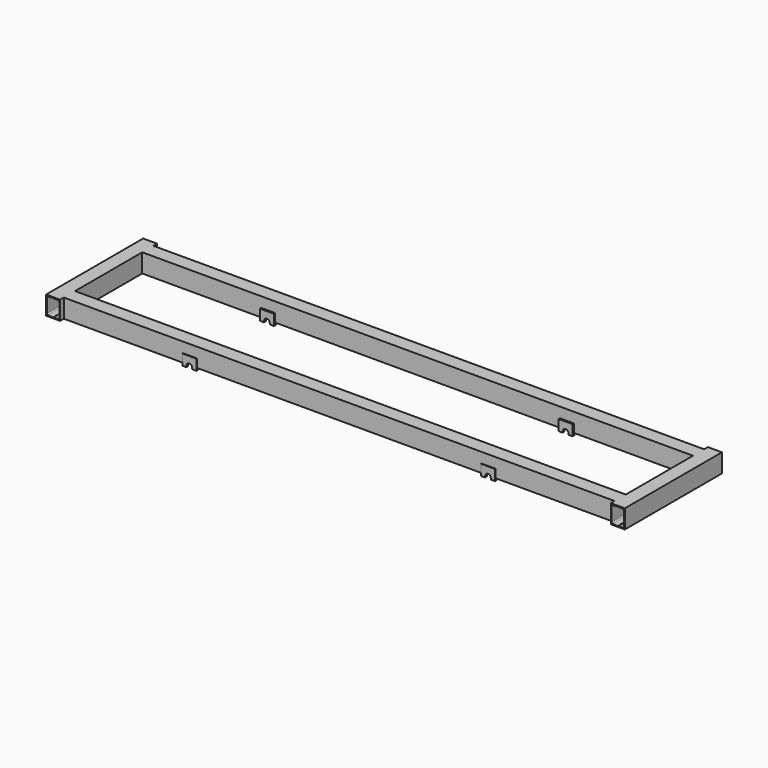
from build123d import *

# Parameters (mm, degrees)
F4_DEPTH       = 3000
F5_W           = 75
F5_H           = 200
F5_W_2         = 50
F5_W_3         = 25
F6_DEPTH       = 1200.001
F8_DEPTH       = 650
F9_W           = 150
F9_H           = 115
F10_DEPTH      = 600
F10_DEPTH_BACK = 600
F11_W          = 370
F11_H          = 130
F11_W_2        = 260
F11_H_2        = 65
F11_W_3        = 110
F11_W_4        = 150
F12_DEPTH      = 50
F13_DEPTH      = 500
F14_DEPTH      = 107.5
F15_DEPTH      = 107.5
F17_DEPTH      = 1257.501
F18_W          = 107.5
F18_H          = 125
F18_W_2        = 42.5
F18_H_2        = 865
F18_H_3        = 82.5
F18_H_4        = 42.5
F18_W_3        = 150
F19_DEPTH      = 115


with BuildPart() as f4:
    # F3 (on Right) → F4 (new body, symmetric)
    with BuildSketch(Plane.YZ):
        with BuildLine():
            ThreePointArc((-530.4770655435, -8.6983562622), (-526.5763359791, -6.7747293194), (-525, -2.7211880737))
            Line((-525, -2.7211880737), (-525, 0))
            Line((-525, 0), (-600, 0))
            Line((-600, 0), (-600, -200))
            Line((-600, -200), (-525, -200))
            Line((-525, -200), (-525, -197.2788119263))
            ThreePointArc((-525, -197.2788119263), (-526.5763359791, -193.2252706806), (-530.4770655435, -191.3016437378))
            Line((-530.4770655435, -191.3016437378), (-586.0229344565, -186.4420099022))
            ThreePointArc((-586.0229344565, -186.4420099022), (-589.9236640209, -184.5183829593), (-591.5, -180.4648417136))
            Line((-591.5, -180.4648417136), (-591.5, -19.5351582864))
            ThreePointArc((-591.5, -19.5351582864), (-589.9236640209, -15.4816170407), (-586.0229344565, -13.5579900978))
            Line((-586.0229344565, -13.5579900978), (-530.4770655435, -8.6983562622))
        make_face()
        with BuildLine():
            Line((-525, 0), (-525, -2.7211880737))
            ThreePointArc((-525, -2.7211880737), (-523.4236640209, -6.7747293194), (-519.5229344565, -8.6983562622))
            Line((-519.5229344565, -8.6983562622), (-463.9770655435, -13.5579900978))
            ThreePointArc((-463.9770655435, -13.5579900978), (-460.0763359791, -15.4816170407), (-458.5, -19.5351582864))
            Line((-458.5, -19.5351582864), (-458.5, -180.4648417136))
            ThreePointArc((-458.5, -180.4648417136), (-460.0763359791, -184.5183829593), (-463.9770655435, -186.4420099022))
            Line((-463.9770655435, -186.4420099022), (-519.5229344565, -191.3016437378))
            ThreePointArc((-519.5229344565, -191.3016437378), (-523.4236640209, -193.2252706806), (-525, -197.2788119263))
            Line((-525, -197.2788119263), (-525, -200))
            Line((-525, -200), (-450, -200))
            Line((-450, -200), (-450, 0))
            Line((-450, 0), (-525, 0))
        make_face()
    extrude(amount=F4_DEPTH, both=True)


with BuildPart() as f4b:
    # F3 (on Right) → F4, piece 2 (new body, symmetric)
    with BuildSketch(Plane.YZ):
        with BuildLine():
            Line((450, -200), (525, -200))
            Line((525, -200), (525, -197.2788119263))
            ThreePointArc((525, -197.2788119263), (523.4236640209, -193.2252706806), (519.5229344565, -191.3016437378))
            Line((519.5229344565, -191.3016437378), (463.9770655435, -186.4420099022))
            ThreePointArc((463.9770655435, -186.4420099022), (460.0763359791, -184.5183829593), (458.5, -180.4648417136))
            Line((458.5, -180.4648417136), (458.5, -19.5351582864))
            ThreePointArc((458.5, -19.5351582864), (460.0763359791, -15.4816170407), (463.9770655435, -13.5579900978))
            Line((463.9770655435, -13.5579900978), (519.5229344565, -8.6983562622))
            ThreePointArc((519.5229344565, -8.6983562622), (523.4236640209, -6.7747293194), (525, -2.7211880737))
            Line((525, -2.7211880737), (525, 0))
            Line((525, 0), (450, 0))
            Line((450, 0), (450, -200))
        make_face()
        with BuildLine():
            Line((525, -197.2788119263), (525, -200))
            Line((525, -200), (600, -200))
            Line((600, -200), (600, 0))
            Line((600, 0), (525, 0))
            Line((525, 0), (525, -2.7211880737))
            ThreePointArc((525, -2.7211880737), (526.5763359791, -6.7747293194), (530.4770655435, -8.6983562622))
            Line((530.4770655435, -8.6983562622), (586.0229344565, -13.5579900978))
            ThreePointArc((586.0229344565, -13.5579900978), (589.9236640209, -15.4816170407), (591.5, -19.5351582864))
            Line((591.5, -19.5351582864), (591.5, -180.4648417136))
            ThreePointArc((591.5, -180.4648417136), (589.9236640209, -184.5183829593), (586.0229344565, -186.4420099022))
            Line((586.0229344565, -186.4420099022), (530.4770655435, -191.3016437378))
            ThreePointArc((530.4770655435, -191.3016437378), (526.5763359791, -193.2252706806), (525, -197.2788119263))
        make_face()
    extrude(amount=F4_DEPTH, both=True)


with BuildPart() as f6_tool:
    # F5 (on face) → F6 (new body, through all)
    with BuildSketch(Plane.XZ.offset(600)):
        with Locations((-3062.5, -100)):
            Rectangle(F5_W, F5_H)
        with Locations((-2975, -100)):
            Rectangle(F5_W_2, F5_H)
        with Locations((3012.5, -100)):
            Rectangle(F5_W_3, F5_H)
        with Locations((2975, -100)):
            Rectangle(F5_W_2, F5_H)
        with Locations((3062.5, -100)):
            Rectangle(F5_W, F5_H)
        with Locations((-3012.5, -100)):
            Rectangle(F5_W_3, F5_H)
    extrude(amount=-F6_DEPTH)


with BuildPart() as f4_1:
    add(f4.part)

    # F6: cut by f6_tool
    add(f6_tool.part, mode=Mode.SUBTRACT)



with BuildPart() as f4b_1:
    add(f4b.part)

    # F6: cut by f6_tool
    add(f6_tool.part, mode=Mode.SUBTRACT)


with BuildPart() as f4_2:
    add(f4_1.part)

    add(f4b_1.part)  # F8 merges F4b
    # F7 (on Front) → F8 (join, symmetric)
    with BuildSketch(Plane.XZ):
        with BuildLine():
            Line((-3100, -200), (-3025, -200))
            Line((-3025, -200), (-3025, -197.2788119263))
            ThreePointArc((-3025, -197.2788119263), (-3026.5763359791, -193.2252706806), (-3030.4770655435, -191.3016437378))
            Line((-3030.4770655435, -191.3016437378), (-3081.0022910416, -186.8812592846))
            ThreePointArc((-3081.0022910416, -186.8812592846), (-3088.4786893733, -183.1943076441), (-3091.5, -175.4250202565))
            Line((-3091.5, -175.4250202565), (-3091.5, -24.5749797435))
            ThreePointArc((-3091.5, -24.5749797435), (-3088.4786893733, -16.8056923559), (-3081.0022910416, -13.1187407154))
            Line((-3081.0022910416, -13.1187407154), (-3030.4770655435, -8.6983562622))
            ThreePointArc((-3030.4770655435, -8.6983562622), (-3026.5763359791, -6.7747293194), (-3025, -2.7211880737))
            Line((-3025, -2.7211880737), (-3025, 0))
            Line((-3025, 0), (-3100, 0))
            Line((-3100, 0), (-3100, -200))
        make_face()
        with BuildLine():
            Line((-3025, -200), (-2950, -200))
            Line((-2950, -200), (-2950, 0))
            Line((-2950, 0), (-3025, 0))
            Line((-3025, 0), (-3025, -2.7211880737))
            ThreePointArc((-3025, -2.7211880737), (-3023.4236640209, -6.7747293194), (-3019.5229344565, -8.6983562622))
            Line((-3019.5229344565, -8.6983562622), (-2968.9977089584, -13.1187407154))
            ThreePointArc((-2968.9977089584, -13.1187407154), (-2961.5213106267, -16.8056923559), (-2958.5, -24.5749797435))
            Line((-2958.5, -24.5749797435), (-2958.5, -175.4250202565))
            ThreePointArc((-2958.5, -175.4250202565), (-2961.5213106267, -183.1943076441), (-2968.9977089584, -186.8812592846))
            Line((-2968.9977089584, -186.8812592846), (-3019.5229344565, -191.3016437378))
            ThreePointArc((-3019.5229344565, -191.3016437378), (-3023.4236640209, -193.2252706806), (-3025, -197.2788119263))
            Line((-3025, -197.2788119263), (-3025, -200))
        make_face()
        with BuildLine():
            Line((3025, -2.7211880737), (3025, 0))
            Line((3025, 0), (2950, 0))
            Line((2950, 0), (2950, -200))
            Line((2950, -200), (3025, -200))
            Line((3025, -200), (3025, -197.2788119263))
            ThreePointArc((3025, -197.2788119263), (3023.4236640209, -193.2252706806), (3019.5229344565, -191.3016437378))
            Line((3019.5229344565, -191.3016437378), (2968.9977089584, -186.8812592846))
            ThreePointArc((2968.9977089584, -186.8812592846), (2961.5213106267, -183.1943076441), (2958.5, -175.4250202565))
            Line((2958.5, -175.4250202565), (2958.5, -24.5749797435))
            ThreePointArc((2958.5, -24.5749797435), (2961.5213106267, -16.8056923559), (2968.9977089584, -13.1187407154))
            Line((2968.9977089584, -13.1187407154), (3019.5229344565, -8.6983562622))
            ThreePointArc((3019.5229344565, -8.6983562622), (3023.4236640209, -6.7747293194), (3025, -2.7211880737))
        make_face()
        with BuildLine():
            Line((3100, 0), (3025, 0))
            Line((3025, 0), (3025, -2.7211880737))
            ThreePointArc((3025, -2.7211880737), (3026.5763359791, -6.7747293194), (3030.4770655435, -8.6983562622))
            Line((3030.4770655435, -8.6983562622), (3081.0022910416, -13.1187407154))
            ThreePointArc((3081.0022910416, -13.1187407154), (3088.4786893733, -16.8056923559), (3091.5, -24.5749797435))
            Line((3091.5, -24.5749797435), (3091.5, -175.4250202565))
            ThreePointArc((3091.5, -175.4250202565), (3088.4786893733, -183.1943076441), (3081.0022910416, -186.8812592846))
            Line((3081.0022910416, -186.8812592846), (3030.4770655435, -191.3016437378))
            ThreePointArc((3030.4770655435, -191.3016437378), (3026.5763359791, -193.2252706806), (3025, -197.2788119263))
            Line((3025, -197.2788119263), (3025, -200))
            Line((3025, -200), (3100, -200))
            Line((3100, -200), (3100, 0))
        make_face()
    extrude(amount=F8_DEPTH, both=True)

    # F9 (on Front) → F10 (cut, two sides)
    with BuildSketch(Plane.XZ) as f10_sk:
        with Locations((-1600, -167.5)):
            Rectangle(F9_W, F9_H)
        with Locations((1600, -167.5)):
            Rectangle(F9_W, F9_H)
    extrude(amount=F10_DEPTH, mode=Mode.SUBTRACT)
    extrude(f10_sk.sketch, amount=-F10_DEPTH_BACK, mode=Mode.SUBTRACT)

    # F11 (on face) → F12 (cut)
    with BuildSketch(Plane(origin=(0, 0, -200), x_dir=(1, 0, 0), z_dir=(0, 0, -1))):
        with Locations((-1600, -525)):
            Rectangle(F11_W, F11_H)
        with Locations((1600, -525)):
            Rectangle(F11_W, F11_H)
        with Locations((-1655, 557.5)):
            Rectangle(F11_W_2, F11_H_2)
        with Locations((-1470, 557.5)):
            Rectangle(F11_W_3, F11_H_2)
        with Locations((-1655, 492.5)):
            Rectangle(F11_W_2, F11_H_2)
        with Locations((-1470, 492.5)):
            Rectangle(F11_W_3, F11_H_2)
        with Locations((1470, 557.5)):
            Rectangle(F11_W_3, F11_H_2)
        with Locations((1600, 557.5)):
            Rectangle(F11_W_4, F11_H_2)
        with Locations((1730, 557.5)):
            Rectangle(F11_W_3, F11_H_2)
        with Locations((1730, 492.5)):
            Rectangle(F11_W_3, F11_H_2)
        with Locations((1600, 492.5)):
            Rectangle(F11_W_4, F11_H_2)
        with Locations((1470, 492.5)):
            Rectangle(F11_W_3, F11_H_2)
    extrude(amount=-F12_DEPTH, mode=Mode.SUBTRACT)


with BuildPart() as f13:
    # F9 (on Front) → F13 (new body, symmetric)
    with BuildSketch(Plane.XZ):
        with Locations((-1600, -167.5)):
            Rectangle(F9_W, F9_H)
    extrude(amount=F13_DEPTH, both=True)

    # F14 (add): a face of the model
    f14_faces = [f13.faces().sort_by_distance(p)[0] for p in [
        (-1600, -500, -167.5),
    ]]
    extrude(f14_faces, amount=F14_DEPTH)


with BuildPart() as f13b:
    # F9 (on Front) → F13, piece 2 (new body, symmetric)
    with BuildSketch(Plane.XZ):
        with Locations((1600, -167.5)):
            Rectangle(F9_W, F9_H)
    extrude(amount=F13_DEPTH, both=True)

    # F14#2 (add): a face of the model
    f14_2_faces = [f13b.faces().sort_by_distance(p)[0] for p in [
        (1600, -500, -167.5),
    ]]
    extrude(f14_2_faces, amount=F14_DEPTH)


with BuildPart() as f15:
    # F15 (new): a face of the model
    f15_faces = [f13b.part.faces().sort_by_distance(p)[0] for p in [
        (1600, 500, -167.5),
    ]]
    extrude(f15_faces, amount=F15_DEPTH)


with BuildPart() as f15b:
    # F15#2 (new): a face of the model
    f15_2_faces = [f13.part.faces().sort_by_distance(p)[0] for p in [
        (-1600, 500, -167.5),
    ]]
    extrude(f15_2_faces, amount=F15_DEPTH)


with BuildPart() as f17_tool:
    # F16 (on face) → F17 (new body, through all)
    with BuildSketch(Plane.XZ.offset(607.5)):
        with BuildLine():
            ThreePointArc((1630, -210), (1600, -180), (1570, -210))
            Line((1570, -210), (1567.5, -225))
            Line((1567.5, -225), (1632.5, -225))
            Line((1632.5, -225), (1630, -210))
        make_face()
        with BuildLine():
            Line((-1567.5, -225), (-1570, -210))
            ThreePointArc((-1570, -210), (-1600, -180), (-1630, -210))
            Line((-1630, -210), (-1632.5, -225))
            Line((-1632.5, -225), (-1567.5, -225))
        make_face()
    extrude(amount=-F17_DEPTH)


with BuildPart() as f13_1:
    add(f13.part)

    # F17: cut by f17_tool
    add(f17_tool.part, mode=Mode.SUBTRACT)


with BuildPart() as f13b_1:
    add(f13b.part)

    # F17: cut by f17_tool
    add(f17_tool.part, mode=Mode.SUBTRACT)


with BuildPart() as f15_1:
    add(f15.part)

    # F17: cut by f17_tool
    add(f17_tool.part, mode=Mode.SUBTRACT)


with BuildPart() as f15b_1:
    add(f15b.part)

    # F17: cut by f17_tool
    add(f17_tool.part, mode=Mode.SUBTRACT)


with BuildPart() as f19_tool:
    # F18 (on face) → F19 (new body, through all)
    with BuildSketch(Plane(origin=(0, 0, -225), x_dir=(1, 0, 0), z_dir=(0, 0, -1))):
        with Locations((-1621.25, 520)):
            Rectangle(F18_W, F18_H)
        with Locations((-1546.25, 520)):
            Rectangle(F18_W_2, F18_H)
        with Locations((-1621.25, 0)):
            Rectangle(F18_W, F18_H_2)
        with Locations((-1546.25, 0)):
            Rectangle(F18_W_2, F18_H_2)
        Polygon((-1675, -582.5), (-1567.5, -582.5), (-1567.5, -500), (-1567.5, -457.5), (-1675, -457.5), align=None)
        with Locations((-1546.25, -541.25)):
            Rectangle(F18_W_2, F18_H_3)
        with Locations((-1546.25, -478.75)):
            Rectangle(F18_W_2, F18_H_4)
        with Locations((1600, 520)):
            Rectangle(F18_W_3, F18_H)
        with Locations((1600, 0)):
            Rectangle(F18_W_3, F18_H_2)
        with Locations((1600, -520)):
            Rectangle(F18_W_3, F18_H)
    extrude(amount=-F19_DEPTH)


with BuildPart() as f13_2:
    add(f13_1.part)

    # F19: cut by f19_tool
    add(f19_tool.part, mode=Mode.SUBTRACT)


with BuildPart() as f13b_2:
    add(f13b_1.part)

    # F19: cut by f19_tool
    add(f19_tool.part, mode=Mode.SUBTRACT)


with BuildPart() as f15_2:
    add(f15_1.part)

    # F19: cut by f19_tool
    add(f19_tool.part, mode=Mode.SUBTRACT)


with BuildPart() as f15b_2:
    add(f15b_1.part)

    # F19: cut by f19_tool
    add(f19_tool.part, mode=Mode.SUBTRACT)


solid = Compound([f4_2.part, f13_2.part, f13b_2.part, f15_2.part, f15b_2.part])
